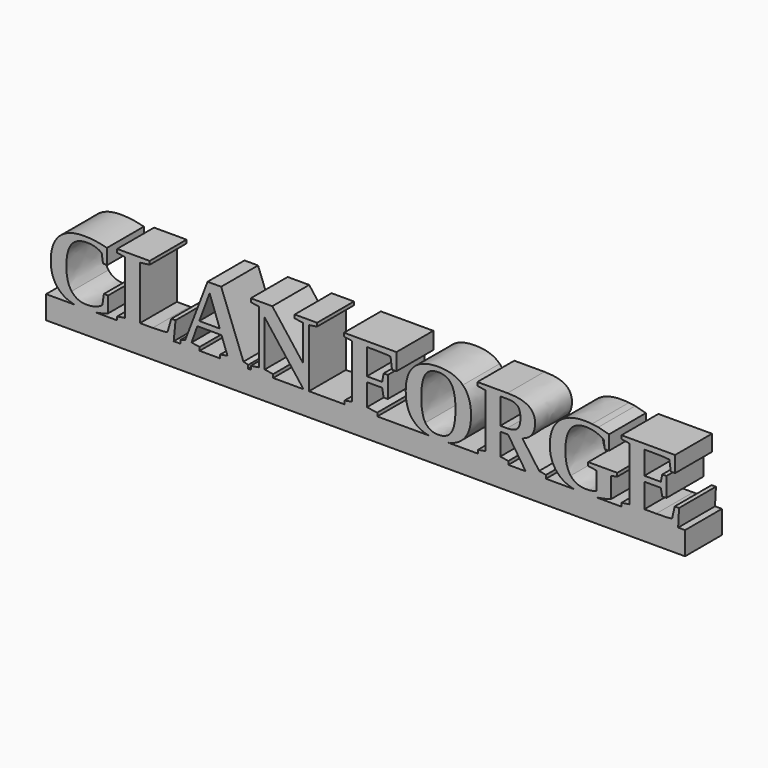
from build123d import *

# Parameters (mm, degrees)
F1_DEPTH = 12.7


with BuildPart() as f1:
    # F0 (on Front) → F1 (new body)
    with BuildSketch(Plane.XZ):
        with BuildLine():
            Line((-68.4216634115, 0.942578125), (-68.4216634115, 0))
            Line((-68.4216634115, 0), (-52.8277832031, 0))
            Line((-52.8277832031, 0), (-52.3358235677, 5.2337890625))
            Line((-52.3358235677, 5.2337890625), (-53.4975097656, 5.2337890625))
            Line((-53.4975097656, 5.2337890625), (-54.555843099, 1.6288411458))
            add(Edge.make_bspline(
                [(-58.603141276, 1.3683919271), (-55.8498209635, 1.3683919271), (-54.555843099, 1.6288411458)],
                knots=[0, 0, 0, 1, 1, 1], degree=2))
            Line((-58.603141276, 1.3683919271), (-62.1295410156, 1.3683919271))
            Line((-62.1295410156, 1.3683919271), (-62.1295410156, 16.0444986979))
            Line((-62.1295410156, 16.0444986979), (-59.4547688802, 16.3834960938))
            Line((-59.4547688802, 16.3834960938), (-59.4547688802, 17.3260742188))
            Line((-59.4547688802, 17.3260742188), (-68.4051269531, 17.3260742188))
            Line((-68.4051269531, 17.3260742188), (-68.4051269531, 16.3834960938))
            Line((-68.4051269531, 16.3834960938), (-66.1975097656, 16.0444986979))
            Line((-66.1975097656, 16.0444986979), (-66.1975097656, 1.2939778646))
            Line((-66.1975097656, 1.2939778646), (-68.4216634115, 0.942578125))
        make_face()
        with BuildLine():
            Line((-52.8277832031, 0), (-68.4216634115, 0))
            Line((-68.4216634115, 0), (-74.343142605, 0))
            add(Edge.make_bspline(
                [(-74.343142605, 0), (-76.0034035409, -0.2604492187), (-77.4505696615, -0.2604492187)],
                knots=[0.0954659663, 0.0954659663, 0.0954659663, 1, 1, 1], degree=2))
            add(Edge.make_bspline(
                [(-77.4505696615, -0.2604492187), (-78.9113372025, -0.2604492187), (-80.1568093662, 0)],
                knots=[0, 0, 0, 0.3355600337, 0.3355600337, 0.3355600337], degree=2))
            Line((-80.1568093662, 0), (-87.9801595052, 0))
            Line((-87.9801595052, 0), (-87.9801595052, -6.35))
            Line((-87.9801595052, -6.35), (87.9801595052, -6.35))
            Line((87.9801595052, -6.35), (87.9801595052, 0))
            Line((87.9801595052, 0), (86.0784667969, 0))
            Line((86.0784667969, 0), (70.4845865885, 0))
            Line((70.4845865885, 0), (63.496240675, 0))
            add(Edge.make_bspline(
                [(63.496240675, 0), (61.6167223735, -0.2604492187), (60.0872884115, -0.2604492187)],
                knots=[0.0954659663, 0.0954659663, 0.0954659663, 1, 1, 1], degree=2))
            add(Edge.make_bspline(
                [(60.0872884115, -0.2604492187), (58.6691944068, -0.2604492187), (57.4309715193, 0)],
                knots=[0, 0, 0, 0.5014947716, 0.5014947716, 0.5014947716], degree=2))
            Line((57.4309715193, 0), (49.6858561198, 0))
            Line((49.6858561198, 0), (44.0799967448, 0))
            Line((44.0799967448, 0), (39.325764974, 0))
            Line((39.325764974, 0), (30.9665852865, 0))
            Line((30.9665852865, 0), (22.8007984266, 0))
            add(Edge.make_bspline(
                [(22.8007984266, 0), (21.5528773482, -0.2604492187), (20.0649251302, -0.2604492187)],
                knots=[0.6610918922, 0.6610918922, 0.6610918922, 1, 1, 1], degree=2))
            add(Edge.make_bspline(
                [(20.0649251302, -0.2604492187), (18.5777401644, -0.2604492187), (17.3291019237, 0)],
                knots=[0, 0, 0, 0.3393724718, 0.3393724718, 0.3393724718], degree=2))
            Line((17.3291019237, 0), (3.2308105469, 0))
            Line((3.2308105469, 0), (-5.7732910156, 0))
            Line((-5.7732910156, 0), (-15.5794108073, 0))
            Line((-15.5794108073, 0), (-17.0924967448, 0))
            Line((-17.0924967448, 0), (-25.4475423177, 0))
            Line((-25.4475423177, 0), (-31.6115071615, 0))
            Line((-31.6115071615, 0), (-32.310172526, 0))
            Line((-32.310172526, 0), (-40.0244303385, 0))
            Line((-40.0244303385, 0), (-45.6923014323, 0))
            Line((-45.6923014323, 0), (-50.963297526, 0))
            Line((-50.963297526, 0), (-52.8277832031, 0))
        make_face()
        with BuildLine():
            add(Edge.make_bspline(
                [(-74.343142605, 0), (-76.0034035409, -0.2604492187), (-77.4505696615, -0.2604492187)],
                knots=[0.0954659663, 0.0954659663, 0.0954659663, 1, 1, 1], degree=2))
            Line((-74.343142605, 0), (-80.1568093662, 0))
            add(Edge.make_bspline(
                [(-77.4505696615, -0.2604492187), (-78.9113372025, -0.2604492187), (-80.1568093662, 0)],
                knots=[0, 0, 0, 0.3355600337, 0.3355600337, 0.3355600337], degree=2))
        make_face()
        with BuildLine():
            Line((-80.1568093662, 0), (-74.343142605, 0))
            add(Edge.make_bspline(
                [(-73.9903157552, 0.0578776042), (-74.1679160147, 0.0274882264), (-74.343142605, 0)],
                knots=[0, 0, 0, 0.0954659663, 0.0954659663, 0.0954659663], degree=2))
            add(Edge.make_bspline(
                [(-70.9641438802, 0.8268229167), (-72.1299641927, 0.3762044271), (-73.9903157552, 0.0578776042)],
                knots=[0, 0, 0, 1, 1, 1], degree=2))
            Line((-70.9641438802, 0.8268229167), (-70.8897298177, 5.2213867187))
            Line((-70.8897298177, 5.2213867187), (-72.0638183594, 5.2213867187))
            Line((-72.0638183594, 5.2213867187), (-72.4772298177, 2.3771158854))
            add(Edge.make_bspline(
                [(-74.1887532552, 1.4593424479), (-73.0973470052, 1.8479492187), (-72.4772298177, 2.3771158854)],
                knots=[0, 0, 0, 1, 1, 1], degree=2))
            add(Edge.make_bspline(
                [(-76.7395019531, 1.0707356771), (-75.2801595052, 1.0707356771), (-74.1887532552, 1.4593424479)],
                knots=[0, 0, 0, 1, 1, 1], degree=2))
            add(Edge.make_bspline(
                [(-80.9521647135, 2.9703613281), (-79.5052246094, 1.0707356771), (-76.7395019531, 1.0707356771)],
                knots=[0, 0, 0, 1, 1, 1], degree=2))
            add(Edge.make_bspline(
                [(-82.3991048177, 8.4997395833), (-82.3991048177, 4.8699869792), (-80.9521647135, 2.9703613281)],
                knots=[0, 0, 0, 1, 1, 1], degree=2))
            add(Edge.make_bspline(
                [(-81.0162434896, 14.2937011719), (-82.3991048177, 12.4271484375), (-82.3991048177, 8.4997395833)],
                knots=[0, 0, 0, 1, 1, 1], degree=2))
            add(Edge.make_bspline(
                [(-76.6361490885, 16.1602539062), (-79.6333821615, 16.1602539062), (-81.0162434896, 14.2937011719)],
                knots=[0, 0, 0, 1, 1, 1], degree=2))
            add(Edge.make_bspline(
                [(-72.6715332031, 14.9985677083), (-74.3747884115, 16.1602539062), (-76.6361490885, 16.1602539062)],
                knots=[0, 0, 0, 1, 1, 1], degree=2))
            Line((-72.6715332031, 14.9985677083), (-72.3077311198, 12.4932942708))
            Line((-72.3077311198, 12.4932942708), (-71.1460449219, 12.4932942708))
            Line((-71.1460449219, 12.4932942708), (-71.224593099, 16.6522135417))
            add(Edge.make_bspline(
                [(-77.4629720052, 17.5203776042), (-74.4533365885, 17.5203776042), (-71.224593099, 16.6522135417)],
                knots=[0, 0, 0, 1, 1, 1], degree=2))
            add(Edge.make_bspline(
                [(-84.3545410156, 15.2135416667), (-82.0229003906, 17.5203776042), (-77.4629720052, 17.5203776042)],
                knots=[0, 0, 0, 1, 1, 1], degree=2))
            add(Edge.make_bspline(
                [(-86.6861816406, 8.4625325521), (-86.6861816406, 12.9067057292), (-84.3545410156, 15.2135416667)],
                knots=[0, 0, 0, 1, 1, 1], degree=2))
            add(Edge.make_bspline(
                [(-84.2449869792, 2.0525878906), (-86.6861816406, 4.365625), (-86.6861816406, 8.4625325521)],
                knots=[0, 0, 0, 1, 1, 1], degree=2))
            add(Edge.make_bspline(
                [(-80.1568093662, 0), (-82.6229596805, 0.5157135915), (-84.2449869792, 2.0525878906)],
                knots=[0.3355600337, 0.3355600337, 0.3355600337, 1, 1, 1], degree=2))
        make_face()
        Polygon((-50.963297526, 0.942578125), (-50.963297526, 0), (-45.6923014323, 0), (-45.6923014323, 0.942578125), (-47.9164550781, 1.2939778646), (-46.3289550781, 5.7753580729), (-39.673030599, 5.7753580729), (-38.0193847656, 1.2939778646), (-40.0244303385, 0.942578125), (-40.0244303385, 0), (-32.310172526, 0), (-32.310172526, 0.942578125), (-33.6289550781, 1.2939778646), (-39.7639811198, 17.4666341146), (-43.5094889323, 17.4666341146), (-49.673453776, 1.2939778646), align=None)
        Polygon((-45.7956542969, 7.1974934896), (-42.9431152344, 14.8580078125), (-40.1649902344, 7.1974934896), align=None, mode=Mode.SUBTRACT)
        Polygon((-31.6115071615, 0.942578125), (-31.6115071615, 0), (-25.4475423177, 0), (-25.4475423177, 0.942578125), (-27.7750488281, 1.2939778646), (-27.7750488281, 13.9278320313), (-17.0924967448, 0), (-15.5794108073, 0), (-15.5794108073, 16.0444986979), (-13.3552571615, 16.3834960938), (-13.3552571615, 17.3260742188), (-19.5192220052, 17.3260742188), (-19.5192220052, 16.3834960938), (-17.1958496094, 16.0444986979), (-17.1958496094, 6.2549153646), (-25.683186849, 17.3260742188), (-31.6115071615, 17.3260742188), (-31.6115071615, 16.3834960938), (-29.3914876302, 16.0444986979), (-29.3914876302, 1.2939778646), align=None)
        with BuildLine():
            Line((70.4845865885, 0), (86.0784667969, 0))
            Line((86.0784667969, 0), (86.3265136719, 4.8327799479))
            Line((86.3265136719, 4.8327799479), (85.1482910156, 4.8327799479))
            Line((85.1482910156, 4.8327799479), (84.4124186198, 1.6288411458))
            add(Edge.make_bspline(
                [(80.0467936198, 1.4221354167), (83.378889974, 1.4221354167), (84.4124186198, 1.6288411458)],
                knots=[0, 0, 0, 1, 1, 1], degree=2))
            Line((80.0467936198, 1.4221354167), (76.7767089844, 1.4221354167))
            Line((76.7767089844, 1.4221354167), (76.7767089844, 8.0987304688))
            Line((76.7767089844, 8.0987304688), (81.3118326823, 8.0987304688))
            Line((81.3118326823, 8.0987304688), (81.7128417969, 6.1350260417))
            Line((81.7128417969, 6.1350260417), (82.862125651, 6.1350260417))
            Line((82.862125651, 6.1350260417), (82.862125651, 11.459765625))
            Line((82.862125651, 11.459765625), (81.7128417969, 11.459765625))
            Line((81.7128417969, 11.459765625), (81.3118326823, 9.5456705729))
            Line((81.3118326823, 9.5456705729), (76.7767089844, 9.5456705729))
            Line((76.7767089844, 9.5456705729), (76.7767089844, 15.9039388021))
            Line((76.7767089844, 15.9039388021), (79.4638834635, 15.9039388021))
            add(Edge.make_bspline(
                [(83.6517415365, 15.7220377604), (82.2048014323, 15.9039388021), (79.4638834635, 15.9039388021)],
                knots=[0, 0, 0, 1, 1, 1], degree=2))
            Line((83.6517415365, 15.7220377604), (84.0651529948, 12.9191080729))
            Line((84.0651529948, 12.9191080729), (85.2392415365, 12.9191080729))
            Line((85.2392415365, 12.9191080729), (85.2392415365, 17.3260742188))
            Line((85.2392415365, 17.3260742188), (70.4845865885, 17.3260742188))
            Line((70.4845865885, 17.3260742188), (70.4845865885, 16.3834960938))
            Line((70.4845865885, 16.3834960938), (72.7087402344, 16.0444986979))
            Line((72.7087402344, 16.0444986979), (72.7087402344, 1.2939778646))
            Line((72.7087402344, 1.2939778646), (70.4845865885, 0.942578125))
            Line((70.4845865885, 0.942578125), (70.4845865885, 0))
        make_face()
        with BuildLine():
            add(Edge.make_bspline(
                [(63.496240675, 0), (61.6167223735, -0.2604492187), (60.0872884115, -0.2604492187)],
                knots=[0.0954659663, 0.0954659663, 0.0954659663, 1, 1, 1], degree=2))
            Line((63.496240675, 0), (57.4309715193, 0))
            add(Edge.make_bspline(
                [(60.0872884115, -0.2604492187), (58.6691944068, -0.2604492187), (57.4309715193, 0)],
                knots=[0, 0, 0, 0.5014947716, 0.5014947716, 0.5014947716], degree=2))
        make_face()
        with BuildLine():
            Line((57.4309715193, 0), (63.496240675, 0))
            add(Edge.make_bspline(
                [(63.896875, 0.0578776042), (63.6946080378, 0.0274882264), (63.496240675, 0)],
                knots=[0, 0, 0, 0.0954659663, 0.0954659663, 0.0954659663], degree=2))
            add(Edge.make_bspline(
                [(67.6196451823, 0.9053710938), (66.015608724, 0.3762044271), (63.896875, 0.0578776042)],
                knots=[0, 0, 0, 1, 1, 1], degree=2))
            Line((67.6196451823, 0.9053710938), (67.6196451823, 6.5360351563))
            Line((67.6196451823, 6.5360351563), (69.3104980469, 6.8750325521))
            Line((69.3104980469, 6.8750325521), (69.3104980469, 7.8300130208))
            Line((69.3104980469, 7.8300130208), (61.3275227865, 7.8300130208))
            Line((61.3275227865, 7.8300130208), (61.3275227865, 6.8750325521))
            Line((61.3275227865, 6.8750325521), (63.5475423177, 6.5360351563))
            Line((63.5475423177, 6.5360351563), (63.5475423177, 1.5254882812))
            add(Edge.make_bspline(
                [(60.6950032552, 1.0707356771), (62.1915527344, 1.0707356771), (63.5475423177, 1.5254882812)],
                knots=[0, 0, 0, 1, 1, 1], degree=2))
            add(Edge.make_bspline(
                [(56.4885416667, 2.9517578125), (57.9416829427, 1.0707356771), (60.6950032552, 1.0707356771)],
                knots=[0, 0, 0, 1, 1, 1], degree=2))
            add(Edge.make_bspline(
                [(55.0354003906, 8.4873372396), (55.0354003906, 4.8327799479), (56.4885416667, 2.9517578125)],
                knots=[0, 0, 0, 1, 1, 1], degree=2))
            add(Edge.make_bspline(
                [(56.4120605469, 14.2875), (55.0354003906, 12.4147460938), (55.0354003906, 8.4873372396)],
                knots=[0, 0, 0, 1, 1, 1], degree=2))
            add(Edge.make_bspline(
                [(60.7983561198, 16.1602539062), (57.7887207031, 16.1602539062), (56.4120605469, 14.2875)],
                knots=[0, 0, 0, 1, 1, 1], degree=2))
            add(Edge.make_bspline(
                [(63.3284342448, 15.7737141927), (62.1006022135, 16.1602539062), (60.7983561198, 16.1602539062)],
                knots=[0, 0, 0, 1, 1, 1], degree=2))
            add(Edge.make_bspline(
                [(65.5773925781, 14.6885091146), (64.556266276, 15.3871744792), (63.3284342448, 15.7737141927)],
                knots=[0, 0, 0, 1, 1, 1], degree=2))
            Line((65.5773925781, 14.6885091146), (65.8874511719, 12.4395507813))
            Line((65.8874511719, 12.4395507813), (67.0491373698, 12.4395507813))
            Line((67.0491373698, 12.4395507813), (67.0491373698, 16.420703125))
            add(Edge.make_bspline(
                [(64.1056477865, 17.1834472656), (64.9076660156, 17.0284179687), (67.0491373698, 16.420703125)],
                knots=[0, 0, 0, 1, 1, 1], degree=2))
            add(Edge.make_bspline(
                [(62.3796549479, 17.4294270833), (63.3036295573, 17.3384765625), (64.1056477865, 17.1834472656)],
                knots=[0, 0, 0, 1, 1, 1], degree=2))
            add(Edge.make_bspline(
                [(60.3312011719, 17.5203776042), (61.4556803385, 17.5203776042), (62.3796549479, 17.4294270833)],
                knots=[0, 0, 0, 1, 1, 1], degree=2))
            add(Edge.make_bspline(
                [(53.2349934896, 15.1680664063), (55.7216634115, 17.5203776042), (60.3312011719, 17.5203776042)],
                knots=[0, 0, 0, 1, 1, 1], degree=2))
            add(Edge.make_bspline(
                [(50.7483235677, 8.4625325521), (50.7483235677, 12.8157552083), (53.2349934896, 15.1680664063)],
                knots=[0, 0, 0, 1, 1, 1], degree=2))
            add(Edge.make_bspline(
                [(51.89140625, 3.7868489583), (50.7483235677, 5.7629557292), (50.7483235677, 8.4625325521)],
                knots=[0, 0, 0, 1, 1, 1], degree=2))
            add(Edge.make_bspline(
                [(55.1470214844, 0.7751464844), (53.0344889323, 1.8107421875), (51.89140625, 3.7868489583)],
                knots=[0, 0, 0, 1, 1, 1], degree=2))
            add(Edge.make_bspline(
                [(57.4309715193, 0), (56.2001300067, 0.2588966119), (55.1470214844, 0.7751464844)],
                knots=[0.5014947716, 0.5014947716, 0.5014947716, 1, 1, 1], degree=2))
        make_face()
        with BuildLine():
            Line((-5.7732910156, 0.942578125), (-5.7732910156, 0))
            Line((-5.7732910156, 0), (3.2308105469, 0))
            Line((3.2308105469, 0), (3.2308105469, 0.942578125))
            Line((3.2308105469, 0.942578125), (0.3493326823, 1.2939778646))
            Line((0.3493326823, 1.2939778646), (0.3493326823, 7.391796875))
            Line((0.3493326823, 7.391796875), (4.5743977865, 7.391796875))
            Line((4.5743977865, 7.391796875), (4.975406901, 5.1676432292))
            Line((4.975406901, 5.1676432292), (6.1246907552, 5.1676432292))
            Line((6.1246907552, 5.1676432292), (6.1246907552, 11.0091471354))
            Line((6.1246907552, 11.0091471354), (4.975406901, 11.0091471354))
            Line((4.975406901, 11.0091471354), (4.5743977865, 8.8097981771))
            Line((4.5743977865, 8.8097981771), (0.3493326823, 8.8097981771))
            Line((0.3493326823, 8.8097981771), (0.3493326823, 15.9039388021))
            Line((0.3493326823, 15.9039388021), (2.4825358073, 15.9039388021))
            add(Edge.make_bspline(
                [(4.7811035156, 15.8584635417), (3.3217610677, 15.9039388021), (2.4825358073, 15.9039388021)],
                knots=[0, 0, 0, 1, 1, 1], degree=2))
            add(Edge.make_bspline(
                [(6.8729654948, 15.7220377604), (6.2404459635, 15.8129882812), (4.7811035156, 15.8584635417)],
                knots=[0, 0, 0, 1, 1, 1], degree=2))
            Line((6.8729654948, 15.7220377604), (7.2863769531, 12.6627929688))
            Line((7.2863769531, 12.6627929688), (8.5018066406, 12.6627929688))
            Line((8.5018066406, 12.6627929688), (8.5018066406, 17.3260742188))
            Line((8.5018066406, 17.3260742188), (-5.9427897135, 17.3260742188))
            Line((-5.9427897135, 17.3260742188), (-5.9427897135, 16.3834960938))
            Line((-5.9427897135, 16.3834960938), (-3.7186360677, 16.0444986979))
            Line((-3.7186360677, 16.0444986979), (-3.7186360677, 1.2939778646))
            Line((-3.7186360677, 1.2939778646), (-5.7732910156, 0.942578125))
        make_face()
        with BuildLine():
            Line((44.0799967448, 0), (49.6858561198, 0))
            Line((49.6858561198, 0), (49.6858561198, 0.942578125))
            Line((49.6858561198, 0.942578125), (47.8131022135, 1.2939778646))
            Line((47.8131022135, 1.2939778646), (43.1870279948, 7.7018554687))
            add(Edge.make_bspline(
                [(46.6762207031, 12.4808919271), (46.6762207031, 8.7601888021), (43.1870279948, 7.7018554687)],
                knots=[0, 0, 0, 1, 1, 1], degree=2))
            add(Edge.make_bspline(
                [(44.7910644531, 16.1499186198), (46.6762207031, 14.9737630208), (46.6762207031, 12.4808919271)],
                knots=[0, 0, 0, 1, 1, 1], degree=2))
            add(Edge.make_bspline(
                [(39.0818522135, 17.3260742188), (42.9059082031, 17.3260742188), (44.7910644531, 16.1499186198)],
                knots=[0, 0, 0, 1, 1, 1], degree=2))
            Line((39.0818522135, 17.3260742188), (30.7970865885, 17.3260742188))
            Line((30.7970865885, 17.3260742188), (30.7970865885, 16.3834960938))
            Line((30.7970865885, 16.3834960938), (33.0212402344, 16.0444986979))
            Line((33.0212402344, 16.0444986979), (33.0212402344, 1.2939778646))
            Line((33.0212402344, 1.2939778646), (30.9665852865, 0.942578125))
            Line((30.9665852865, 0.942578125), (30.9665852865, 0))
            Line((30.9665852865, 0), (39.325764974, 0))
            Line((39.325764974, 0), (39.325764974, 0.942578125))
            Line((39.325764974, 0.942578125), (37.1016113281, 1.2939778646))
            Line((37.1016113281, 1.2939778646), (37.1016113281, 7.3380533854))
            Line((37.1016113281, 7.3380533854), (39.2472167969, 7.3380533854))
            Line((39.2472167969, 7.3380533854), (44.0799967448, 0))
        make_face()
        with BuildLine():
            add(Edge.make_bspline(
                [(42.6454589844, 12.4560872396), (42.6454589844, 14.3908528646), (41.8455078125, 15.1473958333)],
                knots=[0, 0, 0, 1, 1, 1], degree=2))
            add(Edge.make_bspline(
                [(41.806233724, 9.5870117188), (42.6454589844, 10.4138346354), (42.6454589844, 12.4560872396)],
                knots=[0, 0, 0, 1, 1, 1], degree=2))
            add(Edge.make_bspline(
                [(38.978499349, 8.7601888021), (40.9670084635, 8.7601888021), (41.806233724, 9.5870117188)],
                knots=[0, 0, 0, 1, 1, 1], degree=2))
            Line((38.978499349, 8.7601888021), (37.1016113281, 8.7601888021))
            Line((37.1016113281, 8.7601888021), (37.1016113281, 15.9039388021))
            Line((37.1016113281, 15.9039388021), (38.9123535156, 15.9039388021))
            add(Edge.make_bspline(
                [(41.8455078125, 15.1473958333), (41.0455566406, 15.9039388021), (38.9123535156, 15.9039388021)],
                knots=[0, 0, 0, 1, 1, 1], degree=2))
        make_face(mode=Mode.SUBTRACT)
        with BuildLine():
            add(Edge.make_bspline(
                [(17.3291019237, 0), (14.8984840531, 0.5069943438), (13.3717936198, 2.0009114583)],
                knots=[0.3393724718, 0.3393724718, 0.3393724718, 1, 1, 1], degree=2))
            Line((17.3291019237, 0), (22.8007984266, 0))
            add(Edge.make_bspline(
                [(26.7559895833, 2.0071126302), (25.235058593, 0.5080458769), (22.8007984266, 0)],
                knots=[0, 0, 0, 0.6610918922, 0.6610918922, 0.6610918922], degree=2))
            add(Edge.make_bspline(
                [(29.056624349, 8.681640625), (29.056624349, 4.2746744792), (26.7559895833, 2.0071126302)],
                knots=[0, 0, 0, 1, 1, 1], degree=2))
            add(Edge.make_bspline(
                [(26.7828613281, 15.2776204427), (29.056624349, 13.0348632813), (29.056624349, 8.681640625)],
                knots=[0, 0, 0, 1, 1, 1], degree=2))
            add(Edge.make_bspline(
                [(20.0649251302, 17.5203776042), (24.5090983073, 17.5203776042), (26.7828613281, 15.2776204427)],
                knots=[0, 0, 0, 1, 1, 1], degree=2))
            add(Edge.make_bspline(
                [(11.0608235677, 8.681640625), (11.0608235677, 17.5203776042), (20.0649251302, 17.5203776042)],
                knots=[0, 0, 0, 1, 1, 1], degree=2))
            add(Edge.make_bspline(
                [(13.3717936198, 2.0009114583), (11.0608235677, 4.2622721354), (11.0608235677, 8.681640625)],
                knots=[0, 0, 0, 1, 1, 1], degree=2))
        make_face()
        with BuildLine():
            add(Edge.make_bspline(
                [(15.3479003906, 8.681640625), (15.3479003906, 4.5599283854), (16.4785807292, 2.7967285156)],
                knots=[0, 0, 0, 1, 1, 1], degree=2))
            add(Edge.make_bspline(
                [(16.4785807292, 14.4962727865), (15.3479003906, 12.7785481771), (15.3479003906, 8.681640625)],
                knots=[0, 0, 0, 1, 1, 1], degree=2))
            add(Edge.make_bspline(
                [(20.0649251302, 16.2139973958), (17.6092610677, 16.2139973958), (16.4785807292, 14.4962727865)],
                knots=[0, 0, 0, 1, 1, 1], degree=2))
            add(Edge.make_bspline(
                [(23.6347330729, 14.4962727865), (22.5040527344, 16.2139973958), (20.0649251302, 16.2139973958)],
                knots=[0, 0, 0, 1, 1, 1], degree=2))
            add(Edge.make_bspline(
                [(24.7654134115, 8.681640625), (24.7654134115, 12.7785481771), (23.6347330729, 14.4962727865)],
                knots=[0, 0, 0, 1, 1, 1], degree=2))
            add(Edge.make_bspline(
                [(23.6347330729, 2.8029296875), (24.7654134115, 4.5723307292), (24.7654134115, 8.681640625)],
                knots=[0, 0, 0, 1, 1, 1], degree=2))
            add(Edge.make_bspline(
                [(20.0649251302, 1.0335286458), (22.5040527344, 1.0335286458), (23.6347330729, 2.8029296875)],
                knots=[0, 0, 0, 1, 1, 1], degree=2))
            add(Edge.make_bspline(
                [(16.4785807292, 2.7967285156), (17.6092610677, 1.0335286458), (20.0649251302, 1.0335286458)],
                knots=[0, 0, 0, 1, 1, 1], degree=2))
        make_face(mode=Mode.SUBTRACT)
        with BuildLine():
            Line((22.8007984266, 0), (17.3291019237, 0))
            add(Edge.make_bspline(
                [(20.0649251302, -0.2604492187), (18.5777401644, -0.2604492187), (17.3291019237, 0)],
                knots=[0, 0, 0, 0.3393724718, 0.3393724718, 0.3393724718], degree=2))
            add(Edge.make_bspline(
                [(22.8007984266, 0), (21.5528773482, -0.2604492187), (20.0649251302, -0.2604492187)],
                knots=[0.6610918922, 0.6610918922, 0.6610918922, 1, 1, 1], degree=2))
        make_face()
    extrude(amount=F1_DEPTH)


solid = f1.part
